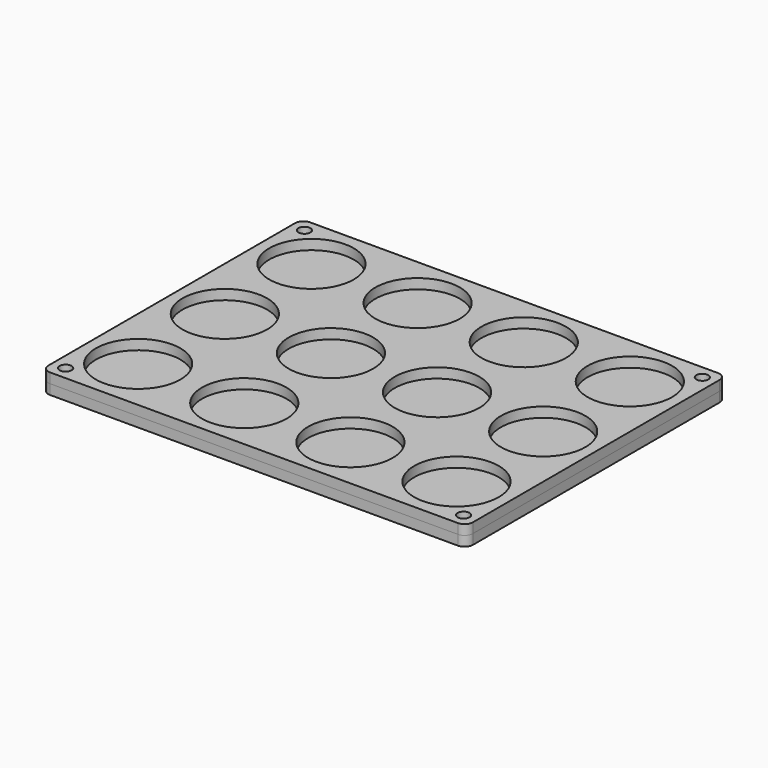
from build123d import *

# Parameters (mm, degrees)
F1_R     = 1.8
F1_R_2   = 12.75
F2_DEPTH = 3
F3_DEPTH = 3
F4_DEPTH = 1
F5_R     = 2.5
F5_2_R   = 2.5


with BuildPart() as f2:
    # F1 (on Top) → F2 (new body)
    with BuildSketch(Plane.XY):
        Polygon((64, 37.2020410289), (64, 49), (52.2020410289, 49), (-54, 49), (-64, 49), (-64, 39), (-64, -39), (-64, -49), (-54, -49), (54, -49), (64, -49), (64, -39), align=None)
        with Locations((-60, -45)):
            Circle(F1_R, mode=Mode.SUBTRACT)
        with Locations((-48, -32.6666666667)):
            Circle(F1_R_2, mode=Mode.SUBTRACT)
        with Locations((-16, -32.6666666667)):
            Circle(F1_R_2, mode=Mode.SUBTRACT)
        with Locations((16, -32.6666666667)):
            Circle(F1_R_2, mode=Mode.SUBTRACT)
        with Locations((60, -45)):
            Circle(F1_R, mode=Mode.SUBTRACT)
        with Locations((48, -32.6666666667)):
            Circle(F1_R_2, mode=Mode.SUBTRACT)
        with Locations((-48, 0)):
            Circle(F1_R_2, mode=Mode.SUBTRACT)
        with Locations((-16, 0)):
            Circle(F1_R_2, mode=Mode.SUBTRACT)
        with Locations((-48, 32.6666666667)):
            Circle(F1_R_2, mode=Mode.SUBTRACT)
        with Locations((-60, 45)):
            Circle(F1_R, mode=Mode.SUBTRACT)
        with Locations((-16, 32.6666666667)):
            Circle(F1_R_2, mode=Mode.SUBTRACT)
        with Locations((16, 0)):
            Circle(F1_R_2, mode=Mode.SUBTRACT)
        with Locations((48, 0)):
            Circle(F1_R_2, mode=Mode.SUBTRACT)
        with Locations((16, 32.6666666667)):
            Circle(F1_R_2, mode=Mode.SUBTRACT)
        with Locations((48, 32.6666666667)):
            Circle(F1_R_2, mode=Mode.SUBTRACT)
        with Locations((60, 45)):
            Circle(F1_R, mode=Mode.SUBTRACT)
    extrude(amount=F2_DEPTH)

    # F5
    f5_edges = [f2.edges().sort_by_distance(p)[0] for p in [
        (-64, 49, 1.5),
        (-64, -49, 1.5),
        (64, -49, 1.5),
        (64, 49, 1.5),
    ]]
    fillet(f5_edges, radius=F5_R)


with BuildPart() as f3:
    # F1 (on Top) → F3 (new body)
    with BuildSketch(Plane.XY):
        Polygon((64, 37.2020410289), (64, 49), (52.2020410289, 49), (-54, 49), (-64, 49), (-64, 39), (-64, -39), (-64, -49), (-54, -49), (54, -49), (64, -49), (64, -39), align=None)
        with Locations((-60, -45)):
            Circle(F1_R, mode=Mode.SUBTRACT)
        with Locations((-48, -32.6666666667)):
            Circle(F1_R_2, mode=Mode.SUBTRACT)
        with Locations((-16, -32.6666666667)):
            Circle(F1_R_2, mode=Mode.SUBTRACT)
        with Locations((16, -32.6666666667)):
            Circle(F1_R_2, mode=Mode.SUBTRACT)
        with Locations((60, -45)):
            Circle(F1_R, mode=Mode.SUBTRACT)
        with Locations((48, -32.6666666667)):
            Circle(F1_R_2, mode=Mode.SUBTRACT)
        with Locations((-48, 0)):
            Circle(F1_R_2, mode=Mode.SUBTRACT)
        with Locations((-16, 0)):
            Circle(F1_R_2, mode=Mode.SUBTRACT)
        with Locations((-48, 32.6666666667)):
            Circle(F1_R_2, mode=Mode.SUBTRACT)
        with Locations((-60, 45)):
            Circle(F1_R, mode=Mode.SUBTRACT)
        with Locations((-16, 32.6666666667)):
            Circle(F1_R_2, mode=Mode.SUBTRACT)
        with Locations((16, 0)):
            Circle(F1_R_2, mode=Mode.SUBTRACT)
        with Locations((48, 0)):
            Circle(F1_R_2, mode=Mode.SUBTRACT)
        with Locations((16, 32.6666666667)):
            Circle(F1_R_2, mode=Mode.SUBTRACT)
        with Locations((48, 32.6666666667)):
            Circle(F1_R_2, mode=Mode.SUBTRACT)
        with Locations((60, 45)):
            Circle(F1_R, mode=Mode.SUBTRACT)
    extrude(amount=-F3_DEPTH)

    # F1 (on Top) → F4 (join)
    with BuildSketch(Plane.XY):
        with Locations((-16, 32.6666666667)):
            Circle(F1_R_2)
        with Locations((-16, 0)):
            Circle(F1_R_2)
        with Locations((-16, -32.6666666667)):
            Circle(F1_R_2)
        with Locations((-48, -32.6666666667)):
            Circle(F1_R_2)
        with Locations((-48, 0)):
            Circle(F1_R_2)
        with Locations((-48, 32.6666666667)):
            Circle(F1_R_2)
        with Locations((16, 32.6666666667)):
            Circle(F1_R_2)
        with Locations((16, 0)):
            Circle(F1_R_2)
        with Locations((16, -32.6666666667)):
            Circle(F1_R_2)
        with Locations((48, 32.6666666667)):
            Circle(F1_R_2)
        with Locations((48, 0)):
            Circle(F1_R_2)
        with Locations((48, -32.6666666667)):
            Circle(F1_R_2)
    extrude(amount=-F4_DEPTH)

    # F5#2
    f5_2_edges = [f3.edges().sort_by_distance(p)[0] for p in [
        (-64, 49, -1.5),
        (-64, -49, -1.5),
        (64, -49, -1.5),
        (64, 49, -1.5),
    ]]
    fillet(f5_2_edges, radius=F5_2_R)


solid = Compound([f2.part, f3.part])
